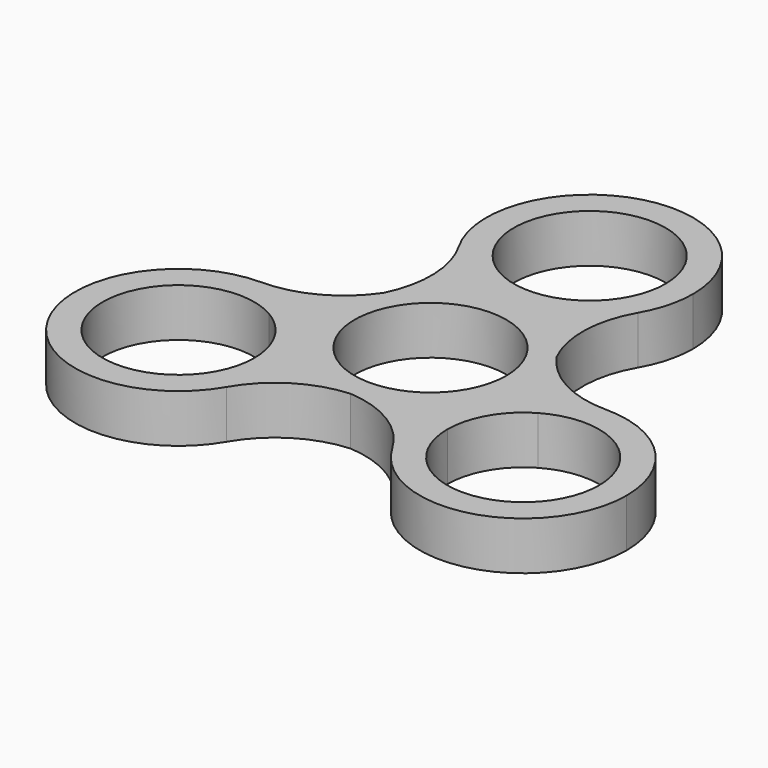
from build123d import *

# Parameters (mm, degrees)
F0_R        = 11
F1_DEPTH    = 7
F2_T1_DEPTH = 7


# Not quite as in the source:
# - a fillet or chamfer that OpenCascade refuses, or shapes differently, is made with other operations: its cross-section is extruded or revolved along the edge and cut away or added


with BuildPart() as f1:
    # F0 (on Top) → F1 (new body)
    with BuildSketch(Plane.XY):
        with BuildLine():
            ThreePointArc((-17.5, -1.443375673), (-37.9903810568, -21.9337567297), (-10, -14.4337567297))
            Line((-10, -14.4337567297), (-14, -14.4337567297))
            ThreePointArc((-14, -14.4337567297), (-34.5262794416, -19.9337567297), (-19.5, -4.9074772881))
            Line((-19.5, -4.9074772881), (-17.5, -1.443375673))
        make_face()
        with BuildLine():
            ThreePointArc((-17.5, -1.443375673), (-12.0096189432, -6.9337567297), (-10, -14.4337567297))
            Line((-10, -14.4337567297), (10, -14.4337567297))
            ThreePointArc((10, -14.4337567297), (12.0096189432, -6.9337567297), (17.5, -1.443375673))
            Line((17.5, -1.443375673), (7.5, 15.8771324027))
            ThreePointArc((7.5, 15.8771324027), (0, 13.8675134595), (-7.5, 15.8771324027))
            Line((-7.5, 15.8771324027), (-17.5, -1.443375673))
        make_face()
        Circle(F0_R, mode=Mode.SUBTRACT)
        with BuildLine():
            Line((-14, -14.4337567297), (-10, -14.4337567297))
            ThreePointArc((-10, -14.4337567297), (-12.0096189432, -6.9337567297), (-17.5, -1.443375673))
            Line((-17.5, -1.443375673), (-19.5, -4.9074772881))
            ThreePointArc((-19.5, -4.9074772881), (-15.4737205584, -8.9337567297), (-14, -14.4337567297))
        make_face()
        with BuildLine():
            ThreePointArc((17.5, -1.443375673), (12.0096189432, -6.9337567297), (10, -14.4337567297))
            Line((10, -14.4337567297), (14, -14.4337567297))
            ThreePointArc((14, -14.4337567297), (15.4737205584, -8.9337567297), (19.5, -4.9074772881))
            Line((19.5, -4.9074772881), (17.5, -1.443375673))
        make_face()
        with BuildLine():
            Line((14, -14.4337567297), (10, -14.4337567297))
            ThreePointArc((10, -14.4337567297), (25, -29.4337567297), (40, -14.4337567297))
            ThreePointArc((40, -14.4337567297), (32.5, -1.443375673), (17.5, -1.443375673))
            Line((17.5, -1.443375673), (19.5, -4.9074772881))
            ThreePointArc((19.5, -4.9074772881), (30.5, -4.9074772881), (36, -14.4337567297))
            ThreePointArc((36, -14.4337567297), (25, -25.4337567297), (14, -14.4337567297))
        make_face()
        with BuildLine():
            ThreePointArc((15, 28.8675134595), (-7.5, 41.8578945162), (-7.5, 15.8771324027))
            Line((-7.5, 15.8771324027), (-5.5, 19.3412340179))
            ThreePointArc((-5.5, 19.3412340179), (-5.5, 38.3937929011), (11, 28.8675134595))
            ThreePointArc((11, 28.8675134595), (9.5262794416, 23.3675134595), (5.5, 19.3412340179))
            Line((5.5, 19.3412340179), (7.5, 15.8771324027))
            ThreePointArc((7.5, 15.8771324027), (12.9903810568, 21.3675134595), (15, 28.8675134595))
        make_face()
        with BuildLine():
            Line((-5.5, 19.3412340179), (-7.5, 15.8771324027))
            ThreePointArc((-7.5, 15.8771324027), (0, 13.8675134595), (7.5, 15.8771324027))
            Line((7.5, 15.8771324027), (5.5, 19.3412340179))
            ThreePointArc((5.5, 19.3412340179), (0, 17.8675134595), (-5.5, 19.3412340179))
        make_face()
    extrude(amount=F1_DEPTH)

    # F2: fillet of radius 15 on 6 edges, made by hand

    # F2_s2 → F2_t1 (join)
    with BuildSketch(Plane.XY):
        with BuildLine():
            ThreePointArc((12.9903810568, 6.3675134595), (10.9807621135, 13.8675134595), (12.9903810568, 21.3675134595))
            ThreePointArc((12.9903810568, 21.3675134595), (10.6066017178, 18.2609117417), (7.5, 15.8771324027))
            Line((7.5, 15.8771324027), (12.9903810568, 6.3675134595))
        make_face()
        with BuildLine():
            ThreePointArc((25, 0.5662432703), (17.5, 2.5758622135), (12.0096189432, 8.0662432703))
            Line((12.0096189432, 8.0662432703), (17.5, -1.443375673))
            ThreePointArc((17.5, -1.443375673), (21.1177143235, 0.0551306646), (25, 0.5662432703))
        make_face()
        with BuildLine():
            ThreePointArc((-12.9903810568, 21.3675134595), (-10.9807621135, 13.8675134595), (-12.9903810568, 6.3675134595))
            Line((-12.9903810568, 6.3675134595), (-7.5, 15.8771324027))
            ThreePointArc((-7.5, 15.8771324027), (-10.6066017178, 18.2609117417), (-12.9903810568, 21.3675134595))
        make_face()
        with BuildLine():
            ThreePointArc((-25, 0.5662432703), (-17.5, 2.5758622135), (-12.0096189432, 8.0662432703))
            Line((-12.0096189432, 8.0662432703), (-17.5, -1.443375673))
            ThreePointArc((-17.5, -1.443375673), (-21.1177143235, 0.0551306646), (-25, 0.5662432703))
        make_face()
        with BuildLine():
            ThreePointArc((-12.0096189432, -21.9337567297), (-6.5192378865, -16.443375673), (0.9807621135, -14.4337567297))
            Line((0.9807621135, -14.4337567297), (-10, -14.4337567297))
            ThreePointArc((-10, -14.4337567297), (-10.5111126057, -18.3160424063), (-12.0096189432, -21.9337567297))
        make_face()
        with BuildLine():
            ThreePointArc((-0.9807621135, -14.4337567297), (6.5192378865, -16.443375673), (12.0096189432, -21.9337567297))
            ThreePointArc((12.0096189432, -21.9337567297), (10.5111126057, -18.3160424063), (10, -14.4337567297))
            Line((10, -14.4337567297), (-0.9807621135, -14.4337567297))
        make_face()
    extrude(amount=F2_T1_DEPTH)


solid = f1.part
